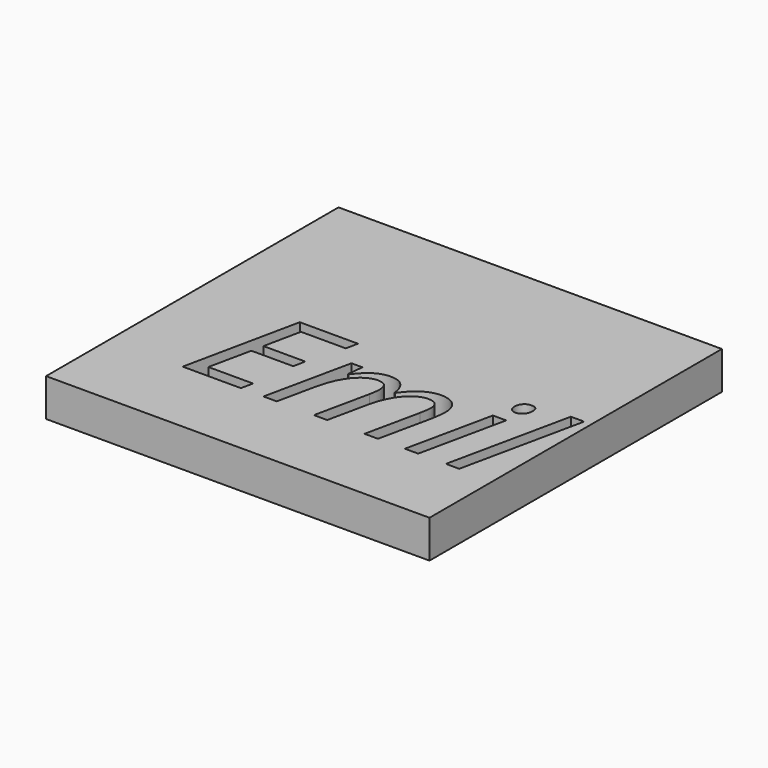
from build123d import *

# Parameters (mm, degrees)
F0_W         = 75.5143761635
F0_H         = 71.9876363873
F1_DEPTH     = 7.4388086796
F2_TEXT_SIZE = 31.9451818036
F3_DEPTH     = 25.4


# Not quite as in the source:
# - Text() gives the source's letters only with a copy of the font that has no kerning and outlines rounded to 1/6400 em; it was checked with that copy


with BuildPart() as f1:
    # F0 (on Top) → F1 (new body)
    with BuildSketch(Plane.XY):
        with Locations((37.7571880817, 35.9938181937)):
            Rectangle(F0_W, F0_H)
    extrude(amount=F1_DEPTH)

    # F2 (on face) → F3 (cut)
    with BuildSketch(Plane.XY.offset(7.4388086796)):
        with Locations((13.0859874763, 15.5889242887)):
            Text('Emil', F2_TEXT_SIZE, font='Open Sans', font_style=FontStyle.ITALIC, text_align=(TextAlign.LEFT, TextAlign.BOTTOM))
    extrude(amount=-F3_DEPTH, mode=Mode.SUBTRACT)


solid = f1.part
